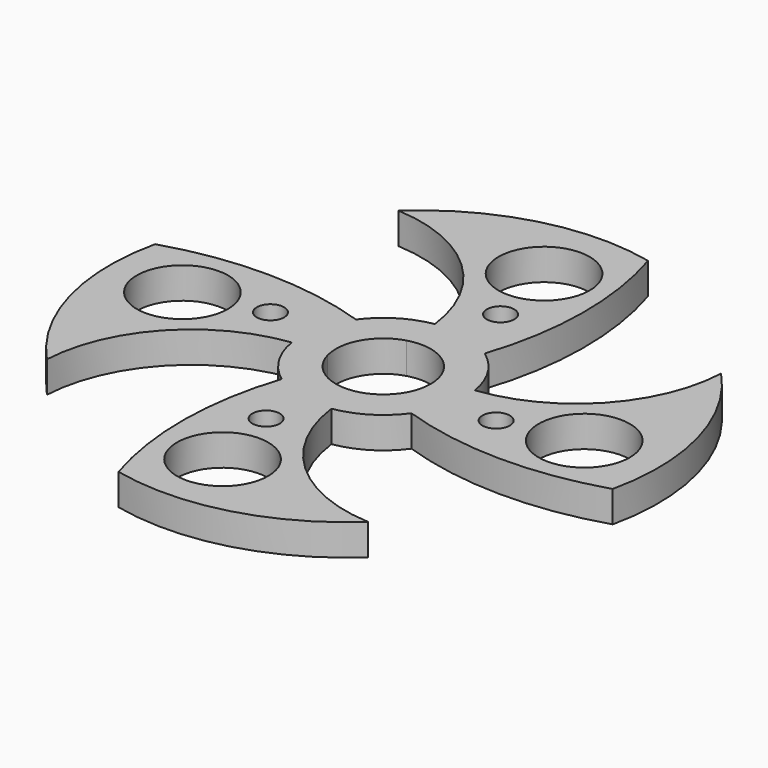
from build123d import *

# Parameters (mm, degrees)
F0_R     = 3.175
F0_R_2   = 10.5664
F1_DEPTH = 7.239


# Not quite as in the source:
# - a feature names something its author has since deleted; it is built from what else it names


with BuildPart() as f1:
    # F0 (on Top) → F1 (new body)
    with BuildSketch(Plane.XY):
        with BuildLine():
            ThreePointArc((49.499110543, 36.0206762632), (40.1908123412, 13.9051845012), (18.8098960555, 3.0150141596))
            ThreePointArc((18.8098960555, 3.0150141596), (18.9898791446, 1.5122797598), (19.05, 0))
            ThreePointArc((19.05, 0), (18.1264129292, -5.8596633283), (15.4452068954, -11.1511472037))
            ThreePointArc((15.4452068954, -11.1511472037), (38.9084897998, -15.0723597821), (62.437543059, -11.5673340383))
            ThreePointArc((62.437543059, -11.5673340383), (61.8751789356, 13.8326514264), (49.499110543, 36.0206762632))
        make_face()
        with Locations((29.21, -3.81)):
            Circle(F0_R, mode=Mode.SUBTRACT)
        with Locations((46.5836, 0)):
            Circle(F0_R_2, mode=Mode.SUBTRACT)
        with BuildLine():
            ThreePointArc((19.05, 0), (18.9898791446, 1.5122797598), (18.8098960555, 3.0150141596))
            ThreePointArc((18.8098960555, 3.0150141596), (16.2245432897, 9.9833208424), (11.1694758624, 15.4319573923))
            ThreePointArc((11.1694758624, 15.4319573923), (4.3764318058, 18.5404785442), (-3.0896344638, 18.7977833502))
            ThreePointArc((-3.0896344638, 18.7977833502), (-9.9628775585, 16.2371047528), (-15.3591721014, 11.2693536797))
            ThreePointArc((-15.3591721014, 11.2693536797), (-18.5170306594, 4.4746033968), (-18.8103206304, -3.0123641517))
            ThreePointArc((-18.8103206304, -3.0123641517), (-16.2548336089, -9.9339259281), (-11.2609801699, -15.3653124151))
            ThreePointArc((-11.2609801699, -15.3653124151), (-4.4663849388, -18.5190147032), (3.0188073829, -18.8092876522))
            ThreePointArc((3.0188073829, -18.8092876522), (9.994585264, -16.2176066483), (15.4452068954, -11.1511472037))
            ThreePointArc((15.4452068954, -11.1511472037), (18.1264129292, -5.8596633283), (19.05, 0))
        make_face()
        with BuildLine():
            ThreePointArc((-3.0490541894, 10.5671032828), (6.6115919208, 8.7890417858), (10.9982, 0))
            ThreePointArc((10.9982, 0), (8.7587082508, -6.6517240635), (2.9522592067, -10.5945537337))
            ThreePointArc((2.9522592067, -10.5945537337), (-5.4079074823, -9.5767917333), (-10.597009287, -2.9434329297))
            ThreePointArc((-10.597009287, -2.9434329297), (-9.601427461, 5.3640464159), (-3.0490541894, 10.5671032828))
        make_face(mode=Mode.SUBTRACT)
        with BuildLine():
            ThreePointArc((-3.0896344638, 18.7977833502), (4.3764318058, 18.5404785442), (11.1694758624, 15.4319573923))
            ThreePointArc((11.1694758624, 15.4319573923), (15.0487096917, 38.8348029597), (11.5431173905, 62.2965262207))
            ThreePointArc((11.5431173905, 62.2965262207), (-13.8155129183, 61.7441471546), (-35.9687104078, 49.3909655905))
            ThreePointArc((-35.9687104078, 49.3909655905), (-13.9597183633, 40.0799728948), (-3.0896344638, 18.7977833502))
        make_face()
        with Locations((0, 46.5836)):
            Circle(F0_R_2, mode=Mode.SUBTRACT)
        with Locations((3.81, 29.21)):
            Circle(F0_R, mode=Mode.SUBTRACT)
        with BuildLine():
            ThreePointArc((35.8851180212, -49.3004770417), (13.913777395, -40.0244664241), (3.0188073829, -18.8092876522))
            ThreePointArc((3.0188073829, -18.8092876522), (-4.4663849388, -18.5190147032), (-11.2609801699, -15.3653124151))
            ThreePointArc((-11.2609801699, -15.3653124151), (-15.1324011861, -38.7568750152), (-11.6267097771, -62.2060376719))
            ThreePointArc((-11.6267097771, -62.2060376719), (13.7319205316, -61.6536586058), (35.8851180212, -49.3004770417))
        make_face()
        with Locations((0, -46.5836)):
            Circle(F0_R_2, mode=Mode.SUBTRACT)
        with Locations((-3.81, -29.21)):
            Circle(F0_R, mode=Mode.SUBTRACT)
        with BuildLine():
            ThreePointArc((-18.8103206304, -3.0123641517), (-18.5170306594, 4.4746033968), (-15.3591721014, 11.2693536797))
            ThreePointArc((-15.3591721014, 11.2693536797), (-38.7496809324, 15.1400454081), (-62.1976706421, 11.6343448498))
            ThreePointArc((-62.1976706421, 11.6343448498), (-61.6452915761, -13.7242854589), (-49.292110012, -35.8774829485))
            ThreePointArc((-49.292110012, -35.8774829485), (-40.0193213234, -13.909615697), (-18.8103206304, -3.0123641517))
        make_face()
        with Locations((-46.5836, 0)):
            Circle(F0_R_2, mode=Mode.SUBTRACT)
        with Locations((-29.21, 3.81)):
            Circle(F0_R, mode=Mode.SUBTRACT)
    extrude(amount=F1_DEPTH)


solid = f1.part
